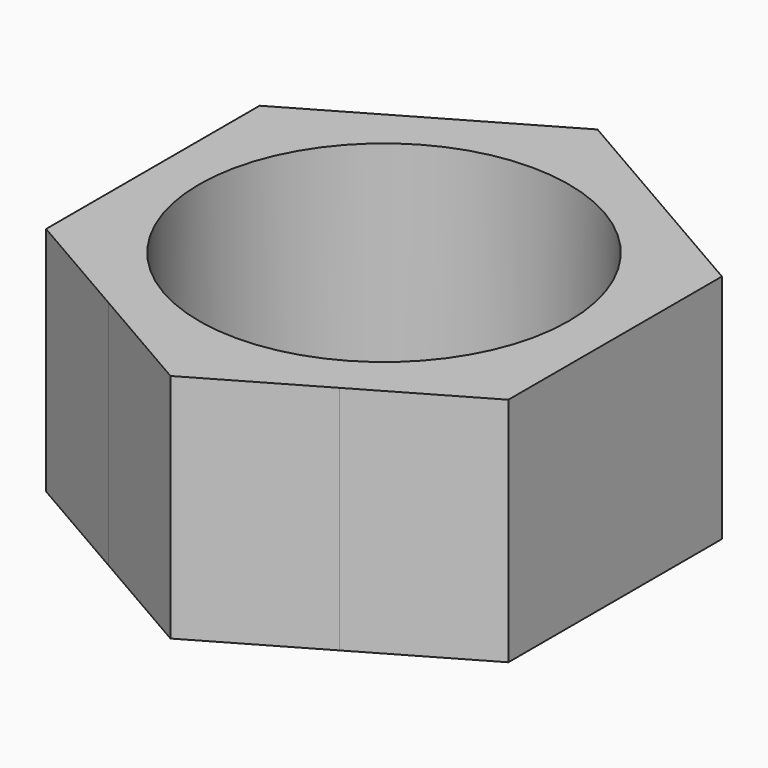
from build123d import *

# Parameters (mm, degrees)
F0_R     = 4
F1_DEPTH = 5


with BuildPart() as f1:
    # F0 (on Top) → F1 (new body)
    with BuildSketch(Plane.XY):
        with BuildLine():
            ThreePointArc((2.499999978, -4.3301270316), (4.3301270126, -2.500000011), (5, 0))
            ThreePointArc((5, 0), (4.330127022, 2.4999999946), (2.5000000107, 4.3301270127))
            ThreePointArc((2.5000000107, 4.3301270127), (-3.05e-08, 5), (-2.5000000636, 4.3301269822))
            ThreePointArc((-2.5000000636, 4.3301269822), (-4.3301270373, 2.4999999682), (-5, 0))
            ThreePointArc((-5, 0), (-4.3301270351, -2.4999999721), (-2.5000000559, -4.3301269867))
            ThreePointArc((-2.5000000559, -4.3301269867), (-4.5e-08, -5), (2.499999978, -4.3301270316))
        make_face()
        Circle(F0_R, mode=Mode.SUBTRACT)
        with BuildLine():
            Line((5, -2.8867513459), (5, 0))
            ThreePointArc((5, 0), (4.3301270126, -2.500000011), (2.499999978, -4.3301270316))
            Line((2.499999978, -4.3301270316), (5, -2.8867513459))
        make_face()
        with BuildLine():
            ThreePointArc((2.5000000107, 4.3301270127), (4.330127022, 2.4999999946), (5, 0))
            Line((5, 0), (5, 2.8867513459))
            Line((5, 2.8867513459), (2.5000000107, 4.3301270127))
        make_face()
        with BuildLine():
            ThreePointArc((-2.5000000636, 4.3301269822), (-3.05e-08, 5), (2.5000000107, 4.3301270127))
            Line((2.5000000107, 4.3301270127), (0, 5.7735026919))
            Line((0, 5.7735026919), (-2.5000000636, 4.3301269822))
        make_face()
        with BuildLine():
            Line((0, -5.7735026919), (2.499999978, -4.3301270316))
            ThreePointArc((2.499999978, -4.3301270316), (-4.5e-08, -5), (-2.5000000559, -4.3301269867))
            Line((-2.5000000559, -4.3301269867), (0, -5.7735026919))
        make_face()
        with BuildLine():
            ThreePointArc((-5, 0), (-4.3301270373, 2.4999999682), (-2.5000000636, 4.3301269822))
            Line((-2.5000000636, 4.3301269822), (-5, 2.8867513459))
            Line((-5, 2.8867513459), (-5, 0))
        make_face()
        with BuildLine():
            Line((-5, -2.8867513459), (-2.5000000559, -4.3301269867))
            ThreePointArc((-2.5000000559, -4.3301269867), (-4.3301270351, -2.4999999721), (-5, 0))
            Line((-5, 0), (-5, -2.8867513459))
        make_face()
    extrude(amount=F1_DEPTH)


solid = f1.part
